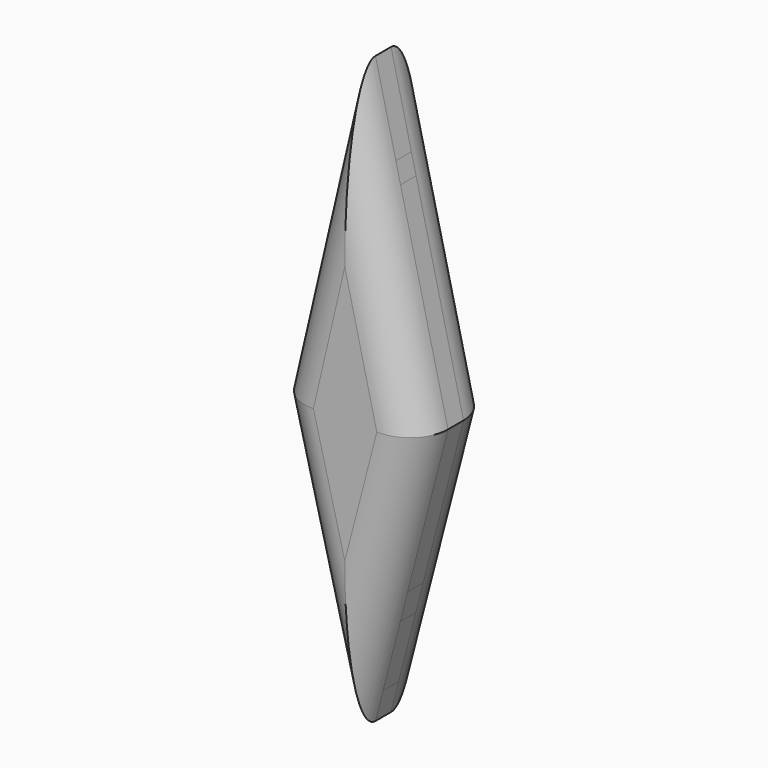
from build123d import *

# Parameters (mm, degrees)
F1_DEPTH    = 6.35
F2_DEPTH    = 6.35
F4_DEPTH    = 25.4
F5_T1_DEPTH = 66.3794734437
F5_T3_DEPTH = 66.4252991911
F5_T5_DEPTH = 63.2525240866
F5_T7_DEPTH = 63.2028524021


# Not quite as in the source:
# - a fillet or chamfer that OpenCascade refuses, or shapes differently, is made with other operations: its cross-section is extruded or revolved along the edge and cut away or added


with BuildPart() as f1:
    # F0 (on Front) → F1 (new body)
    with BuildSketch(Plane.XZ):
        Polygon((10.5009634349, -8.6313571018), (0, -8.4001217037), (-10.5245159939, -8.168367669), (-8.3013391122, -91.856867075), (8.6683045514, -91.856867075), align=None)
    extrude(amount=F1_DEPTH)

    # F2 (add): a face of the model
    f2_faces = [f1.faces().sort_by_distance(p)[0] for p in [
        (0.0745348421, 0, -48.6438367355),
    ]]
    extrude(f2_faces, amount=F2_DEPTH)

    # F3 (on face) → F4 (cut)
    with BuildSketch(Plane.XZ.offset(6.35)):
        Polygon((7.741477061, -8.5705921125), (0, -12.6956291497), (-8.4089043082, -8.2149542811), (-10.5245159939, -8.168367669), (-10.4707083295, -10.1938847244), (0, -15.2933746576), (10.4665109394, -10.1959289555), (10.5009634349, -8.6313571018), align=None)
        Polygon((-8.4089043082, -8.2149542811), (0, -12.6956291497), (7.741477061, -8.5705921125), align=None)
        Polygon((0, -15.2933746576), (-10.4707083295, -10.1938847244), (-10.1647846318, -21.7099702861), (-2.6734457948, -26.4930181658), (-2.660532576, -26.5012629595), (-2.6115273083, -26.532551698), align=None)
        Polygon((10.2136542458, -21.6787681594), (10.4665109394, -10.1959289555), (0, -15.2933746576), (2.660532576, -26.5012629595), align=None)
        Polygon((-2.6734457948, -26.4930181658), (-10.1647846318, -21.7099702861), (-10.0923027152, -24.4384544155), (-3.4606218927, -28.9392464633), (-3.2699760565, -29.068634063), (-3.2102312503, -29.1091816943), (-2.6115273083, -26.532551698), (-2.660532576, -26.5012629595), align=None)
        Polygon((10.15380398, -24.3967147102), (10.2136542458, -21.6787681594), (2.660532576, -26.5012629595), (3.2699760565, -29.068634063), align=None)
        Polygon((-3.4606218927, -28.9392464633), (-10.0923027152, -24.4384544155), (-9.2748739024, -55.2094611118), (-3.2102312503, -29.1091816943), (-3.2699760565, -29.068634063), align=None)
        Polygon((9.4752950296, -55.2094611118), (10.15380398, -24.3967147102), (3.2699760565, -29.068634063), align=None)
        Polygon((-4.0967862529, -75.6694136894), (-9.2748739024, -55.2094611118), (-8.7972565245, -73.1887240187), (-4.2695118804, -75.5782571337), (-4.199302435, -75.6153104147), align=None)
        Polygon((9.0827017549, -73.0380792973), (9.4752950296, -55.2094611118), (4.199302435, -75.6153104147), align=None)
        Polygon((-3.1505538377, -79.4082206875), (-4.0967862529, -75.6694136894), (-4.199302435, -75.6153104147), (-4.2695118804, -75.5782571337), (-8.7972565245, -73.1887240187), (-8.7198462703, -76.1027287805), (-3.3105833326, -79.3132398248), (-3.2309755221, -79.3604887305), align=None)
        Polygon((9.0827017549, -73.0380792973), (4.199302435, -75.6153104147), (3.2309755221, -79.3604887305), (9.0191284413, -75.9250985328), align=None)
        Polygon((-0.965611629, -88.0414878319), (-3.1505538377, -79.4082206875), (-3.2309755221, -79.3604887305), (-3.3105833326, -79.3132398248), (-8.7198462703, -76.1027287805), (-8.5424459568, -82.7807246478), (-1.0061214638, -88.0133609601), (-0.9910429813, -88.023830283), align=None)
        Polygon((9.0191284413, -75.9250985328), (3.2309755221, -79.3604887305), (0.9910429813, -88.023830283), (8.8732221424, -82.5510594467), align=None)
        Polygon((0, -91.856867075), (-0.965611629, -88.0414878319), (-0.9910429813, -88.023830283), (-1.0061214638, -88.0133609601), (-8.5424459568, -82.7807246478), (-8.434321605, -86.8509202434), align=None)
        Polygon((8.8732221424, -82.5510594467), (0.9910429813, -88.023830283), (0, -91.856867075), (8.7830958233, -86.6439154273), align=None)
        Polygon((-8.3013391122, -91.856867075), (0, -91.856867075), (-8.434321605, -86.8509202434), align=None)
        Polygon((8.7830958233, -86.6439154273), (0, -91.856867075), (8.6683045514, -91.856867075), align=None)
    extrude(amount=-F4_DEPTH, mode=Mode.SUBTRACT)

    # F5: fillet of radius 5.08 on 8 edges, made by hand

    # F5_s2 → F5_t1 (cut)
    with BuildSketch(Plane(origin=(-15.5207879816, 0, -66.796500031), x_dir=(0, 1, 0), z_dir=(0.2263297481, 0, 0.9740507405))):
        with BuildLine():
            ThreePointArc((-6.35, -8.5413456341), (-4.8621024484, -4.9492431857), (-1.27, -3.4613456341))
            Line((-1.27, -3.4613456341), (-6.35, -3.4613456341))
            Line((-6.35, -3.4613456341), (-6.35, -8.5413456341))
        make_face()
        with BuildLine():
            ThreePointArc((6.35, -8.5413456341), (4.8621024484, -4.9492431857), (1.27, -3.4613456341))
            Line((1.27, -3.4613456341), (6.35, -3.4613456341))
            Line((6.35, -3.4613456341), (6.35, -8.5413456341))
        make_face()
    extrude(amount=F5_T1_DEPTH, mode=Mode.SUBTRACT)

    # F5_s4 → F5_t3 (cut)
    with BuildSketch(Plane(origin=(0.5034707355, 0, -2.1209451889), x_dir=(0, 1, 0), z_dir=(0.2309622408, 0, -0.9729627143))):
        with BuildLine():
            ThreePointArc((-1.27, -3.5321920799), (-4.8621024484, -5.0200896315), (-6.35, -8.6121920799))
            Line((-6.35, -8.6121920799), (-6.35, -3.5321920799))
            Line((-6.35, -3.5321920799), (-1.27, -3.5321920799))
        make_face()
        with BuildLine():
            ThreePointArc((1.27, -3.5321920799), (4.8621024484, -5.0200896315), (6.35, -8.6121920799))
            Line((6.35, -8.6121920799), (6.35, -3.5321920799))
            Line((6.35, -3.5321920799), (1.27, -3.5321920799))
        make_face()
    extrude(amount=F5_T3_DEPTH, mode=Mode.SUBTRACT)

    # F5_s6 → F5_t5 (cut)
    with BuildSketch(Plane(origin=(-9.6073030151, 0, -37.1579705651), x_dir=(0, 1, 0), z_dir=(-0.2503213526, 0, -0.9681628068))):
        with BuildLine():
            ThreePointArc((-6.35, 17.9137352141), (-4.8621024484, 21.5058376626), (-1.27, 22.9937352141))
            Line((-1.27, 22.9937352141), (-6.35, 22.9937352141))
            Line((-6.35, 22.9937352141), (-6.35, 17.9137352141))
        make_face()
        with BuildLine():
            ThreePointArc((1.27, 22.9937352141), (4.8621024484, 21.5058376626), (6.35, 17.9137352141))
            Line((6.35, 17.9137352141), (6.35, 22.9937352141))
            Line((6.35, 22.9937352141), (1.27, 22.9937352141))
        make_face()
    extrude(amount=F5_T5_DEPTH, mode=Mode.SUBTRACT)

    # F5_s8 → F5_t7 (cut)
    with BuildSketch(Plane(origin=(24.9640295189, 0, -98.6392843591), x_dir=(0, 1, 0), z_dir=(-0.2453485204, 0, 0.9694349403))):
        with BuildLine():
            ThreePointArc((-6.35, 17.4569464222), (-4.8621024484, 21.0490488706), (-1.27, 22.5369464222))
            Line((-1.27, 22.5369464222), (-6.35, 22.5369464222))
            Line((-6.35, 22.5369464222), (-6.35, 17.4569464222))
        make_face()
        with BuildLine():
            ThreePointArc((6.35, 17.4569464222), (4.8621024484, 21.0490488706), (1.27, 22.5369464222))
            Line((1.27, 22.5369464222), (6.35, 22.5369464222))
            Line((6.35, 22.5369464222), (6.35, 17.4569464222))
        make_face()
    extrude(amount=F5_T7_DEPTH, mode=Mode.SUBTRACT)


solid = f1.part
